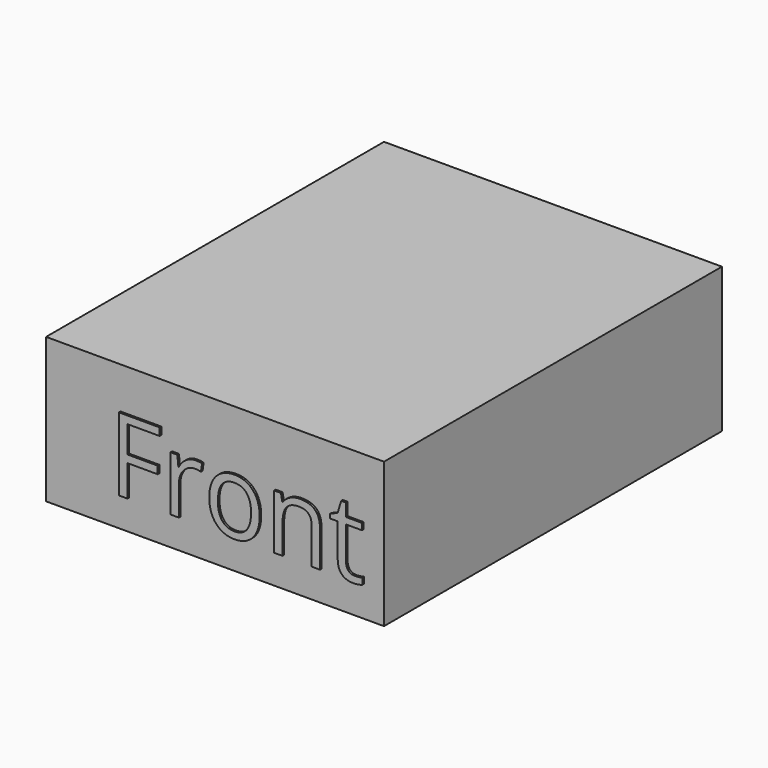
from build123d import *

# Parameters (mm, degrees)
F0_W         = 4267.2
F0_H         = 5334
F1_DEPTH     = 1828.8
F2_TEXT_SIZE = 1293.4330022997
F3_DEPTH     = 25.4


# Not quite as in the source:
# - Text() gives the source's letters only with a copy of the font that has no kerning and outlines rounded to 1/6400 em; it was checked with that copy


with BuildPart() as f1:
    # F0 (on Top) → F1 (new body)
    with BuildSketch(Plane.XY):
        Rectangle(F0_W, F0_H)
    extrude(amount=F1_DEPTH)

    # F2 (on face) → F3 (join)
    with BuildSketch(Plane.XZ.offset(2667)):
        with Locations((-1320.6313848495, 381.7830383778)):
            Text('Front', F2_TEXT_SIZE, font='Open Sans', text_align=(TextAlign.LEFT, TextAlign.BOTTOM))
    extrude(amount=F3_DEPTH)


solid = f1.part
